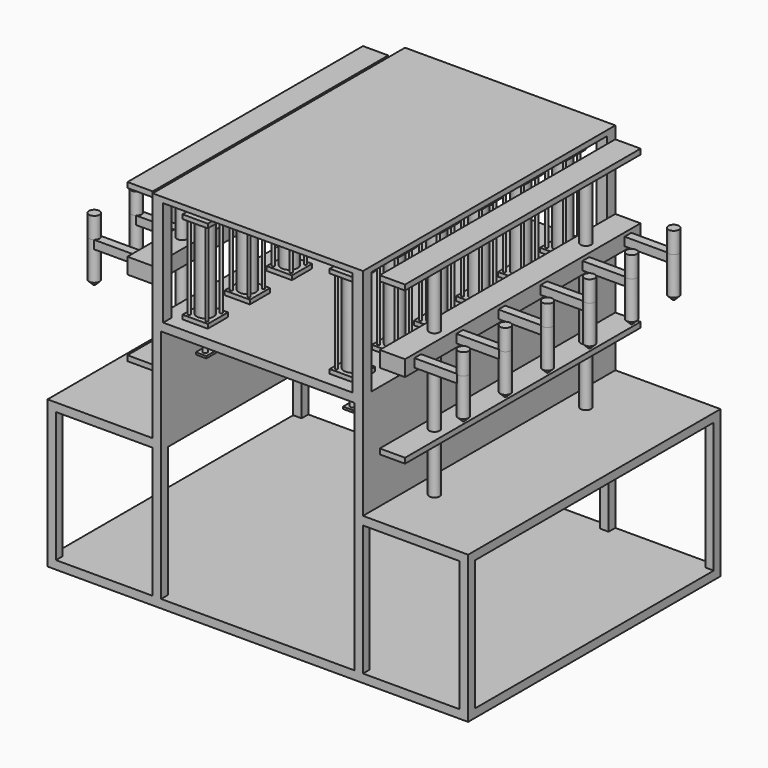
from build123d import *

# Parameters (mm, degrees)
F1_DEPTH       = 1500
F2_W           = 460
F2_H           = 620
F3_DEPTH       = 1500.001
F4_W           = 1420
F4_H           = 620
F5_DEPTH       = 2000.001
F6_W           = 120
F6_H           = 120
F7_DEPTH       = 20
F8_R           = 40
F9_DEPTH       = 400
F10_R          = 6
F11_DEPTH      = 400
F12_W          = 120
F12_H          = 120
F13_DEPTH      = 20
F14_R          = 11
F15_DEPTH      = 100
F16_W          = 50
F16_H          = 1300
F17_DEPTH      = 10
F18_R          = 25
F19_DEPTH      = 1000
F21_W          = 120
F21_H          = 1400
F22_DEPTH      = 25
F23_W          = 120
F23_H          = 1400
F24_DEPTH      = 25
F26_W          = 120
F26_H          = 1400
F27_DEPTH      = 75
F28_W          = 40
F28_H          = 40
F29_DEPTH      = 217.5
F30_R          = 25
F31_DEPTH      = 100
F31_DEPTH_BACK = 200
F32_SIZE       = 20
F33_W          = 50
F33_H          = 50
F34_DEPTH      = 500
F35_W          = 1000
F35_H          = 1500
F36_DEPTH      = 25


# Not quite as in the source:
# - a pattern or mirror of a feature is missing from the dataset's text; its kind, count and spacing are read off the source's solid


with BuildPart() as f1:
    # F0 (on Front) → F1 (new body)
    with BuildSketch(Plane.XZ):
        Polygon((-1000, 0), (0, 0), (0, 1200), (-500, 1200), (-500, 700), (-1000, 700), align=None)
        Polygon((0, 1200), (0, 0), (1000, 0), (1000, 700), (500, 700), (500, 1200), align=None)
    extrude(amount=F1_DEPTH)

    # F2 (on face) → F3 (cut, through all)
    with BuildSketch(Plane.XZ.offset(1500)):
        with Locations((-730, 350)):
            Rectangle(F2_W, F2_H)
        with Locations((730, 350)):
            Rectangle(F2_W, F2_H)
        Polygon((460, 1160), (-460, 1160), (-460, 660), (-460, 40), (460, 40), (460, 660), align=None)
    extrude(amount=-F3_DEPTH, mode=Mode.SUBTRACT)

    # F4 (on face) → F5 (cut, through all)
    with BuildSketch(Plane.YZ.offset(1000)):
        with Locations((-750, 350)):
            Rectangle(F4_W, F4_H)
    extrude(amount=-F5_DEPTH, mode=Mode.SUBTRACT)

    # F6 (on face) → F7 (join)
    with BuildSketch(Plane.XY.offset(1200)):
        with Locations((-350, -125)):
            Rectangle(F6_W, F6_H)
        with Locations((-350, -375)):
            Rectangle(F6_W, F6_H)
        with Locations((-350, -625)):
            Rectangle(F6_W, F6_H)
        with Locations((-350, -875)):
            Rectangle(F6_W, F6_H)
        with Locations((-350, -1125)):
            Rectangle(F6_W, F6_H)
        with Locations((-350, -1375)):
            Rectangle(F6_W, F6_H)
        with Locations((350, -125)):
            Rectangle(F6_W, F6_H)
        with Locations((350, -375)):
            Rectangle(F6_W, F6_H)
        with Locations((350, -625)):
            Rectangle(F6_W, F6_H)
        with Locations((350, -875)):
            Rectangle(F6_W, F6_H)
        with Locations((350, -1125)):
            Rectangle(F6_W, F6_H)
        with Locations((350, -1375)):
            Rectangle(F6_W, F6_H)
    extrude(amount=F7_DEPTH)

    # F8 (on face) → F9 (join)
    with BuildSketch(Plane.XY.offset(1220)):
        with Locations((-350, -1375)):
            Circle(F8_R)
        with Locations((-350, -1125)):
            Circle(F8_R)
        with Locations((-350, -875)):
            Circle(F8_R)
        with Locations((-350, -625)):
            Circle(F8_R)
        with Locations((-350, -375)):
            Circle(F8_R)
        with Locations((-350, -125)):
            Circle(F8_R)
        with Locations((350, -1375)):
            Circle(F8_R)
        with Locations((350, -1125)):
            Circle(F8_R)
        with Locations((350, -875)):
            Circle(F8_R)
        with Locations((350, -625)):
            Circle(F8_R)
        with Locations((350, -375)):
            Circle(F8_R)
        with Locations((350, -125)):
            Circle(F8_R)
    extrude(amount=F9_DEPTH)

    # F10 (on face) → F11 (join)
    with BuildSketch(Plane.XY.offset(1220)):
        with Locations((-307.5, -1332.5)):
            Circle(F10_R)
        with Locations((-392.5, -1332.5)):
            Circle(F10_R)
        with Locations((-307.5, -1417.5)):
            Circle(F10_R)
        with Locations((-392.5, -1417.5)):
            Circle(F10_R)
        with Locations((-307.5, -1082.5)):
            Circle(F10_R)
        with Locations((-392.5, -1082.5)):
            Circle(F10_R)
        with Locations((-392.5, -1167.5)):
            Circle(F10_R)
        with Locations((-307.5, -1167.5)):
            Circle(F10_R)
        with Locations((-307.5, -832.5)):
            Circle(F10_R)
        with Locations((-392.5, -832.5)):
            Circle(F10_R)
        with Locations((-392.5, -917.5)):
            Circle(F10_R)
        with Locations((-307.5, -917.5)):
            Circle(F10_R)
        with Locations((-307.5, -582.5)):
            Circle(F10_R)
        with Locations((-392.5, -582.5)):
            Circle(F10_R)
        with Locations((-392.5, -667.5)):
            Circle(F10_R)
        with Locations((-307.5, -667.5)):
            Circle(F10_R)
        with Locations((-307.5, -332.5)):
            Circle(F10_R)
        with Locations((-392.5, -332.5)):
            Circle(F10_R)
        with Locations((-392.5, -417.5)):
            Circle(F10_R)
        with Locations((-307.5, -417.5)):
            Circle(F10_R)
        with Locations((-307.5, -82.5)):
            Circle(F10_R)
        with Locations((-392.5, -82.5)):
            Circle(F10_R)
        with Locations((-392.5, -167.5)):
            Circle(F10_R)
        with Locations((-307.5, -167.5)):
            Circle(F10_R)
        with Locations((392.5, -1332.5)):
            Circle(F10_R)
        with Locations((307.5, -1332.5)):
            Circle(F10_R)
        with Locations((307.5, -1417.5)):
            Circle(F10_R)
        with Locations((392.5, -1417.5)):
            Circle(F10_R)
        with Locations((392.5, -1082.5)):
            Circle(F10_R)
        with Locations((307.5, -1082.5)):
            Circle(F10_R)
        with Locations((307.5, -1167.5)):
            Circle(F10_R)
        with Locations((392.5, -1167.5)):
            Circle(F10_R)
        with Locations((392.5, -832.5)):
            Circle(F10_R)
        with Locations((307.5, -832.5)):
            Circle(F10_R)
        with Locations((307.5, -917.5)):
            Circle(F10_R)
        with Locations((392.5, -917.5)):
            Circle(F10_R)
        with Locations((392.5, -582.5)):
            Circle(F10_R)
        with Locations((307.5, -582.5)):
            Circle(F10_R)
        with Locations((307.5, -667.5)):
            Circle(F10_R)
        with Locations((392.5, -667.5)):
            Circle(F10_R)
        with Locations((392.5, -332.5)):
            Circle(F10_R)
        with Locations((307.5, -332.5)):
            Circle(F10_R)
        with Locations((307.5, -417.5)):
            Circle(F10_R)
        with Locations((392.5, -417.5)):
            Circle(F10_R)
        with Locations((392.5, -82.5)):
            Circle(F10_R)
        with Locations((307.5, -82.5)):
            Circle(F10_R)
        with Locations((307.5, -167.5)):
            Circle(F10_R)
        with Locations((392.5, -167.5)):
            Circle(F10_R)
    extrude(amount=F11_DEPTH)

    # F12 (on face) → F13 (join)
    with BuildSketch(Plane.XY.offset(1620)):
        with Locations((-350, -1375)):
            Rectangle(F12_W, F12_H)
        with Locations((-350, -1125)):
            Rectangle(F12_W, F12_H)
        with Locations((-350, -875)):
            Rectangle(F12_W, F12_H)
        with Locations((-350, -625)):
            Rectangle(F12_W, F12_H)
        with Locations((-350, -375)):
            Rectangle(F12_W, F12_H)
        with Locations((-350, -125)):
            Rectangle(F12_W, F12_H)
        with Locations((350, -1375)):
            Rectangle(F12_W, F12_H)
        with Locations((350, -1125)):
            Rectangle(F12_W, F12_H)
        with Locations((350, -875)):
            Rectangle(F12_W, F12_H)
        with Locations((350, -625)):
            Rectangle(F12_W, F12_H)
        with Locations((350, -375)):
            Rectangle(F12_W, F12_H)
        with Locations((350, -125)):
            Rectangle(F12_W, F12_H)
    extrude(amount=F13_DEPTH)

    # F14 (on face) → F15 (join)
    with BuildSketch(Plane(origin=(0, 0, 1160), x_dir=(1, 0, 0), z_dir=(0, 0, -1))):
        with Locations((-350, 125)):
            Circle(F14_R)
        with Locations((-350, 375)):
            Circle(F14_R)
        with Locations((-350, 625)):
            Circle(F14_R)
        with Locations((-350, 875)):
            Circle(F14_R)
        with Locations((-350, 1125)):
            Circle(F14_R)
        with Locations((-350, 1375)):
            Circle(F14_R)
        with Locations((350, 125)):
            Circle(F14_R)
        with Locations((350, 375)):
            Circle(F14_R)
        with Locations((350, 625)):
            Circle(F14_R)
        with Locations((350, 875)):
            Circle(F14_R)
        with Locations((350, 1125)):
            Circle(F14_R)
        with Locations((350, 1375)):
            Circle(F14_R)
    extrude(amount=F15_DEPTH)

    # F16 (on face) → F17 (join)
    with BuildSketch(Plane(origin=(0, 0, 1060), x_dir=(1, 0, 0), z_dir=(0, 0, -1))):
        with Locations((-350, 750)):
            Rectangle(F16_W, F16_H)
        with Locations((350, 750)):
            Rectangle(F16_W, F16_H)
    extrude(amount=F17_DEPTH)

    # F18 (on face) → F19 (join)
    with BuildSketch(Plane.XY.offset(700)):
        with Locations((-600, -300)):
            Circle(F18_R)
        with Locations((600, -300)):
            Circle(F18_R)
        with Locations((-600, -1200)):
            Circle(F18_R)
        with Locations((600, -1200)):
            Circle(F18_R)
    extrude(amount=F19_DEPTH)

    # F21 (on offset) → F22 (join)
    with BuildSketch(Plane.XY.offset(950)):
        with Locations((-600, -750)):
            Rectangle(F21_W, F21_H)
        with Locations((600, -750)):
            Rectangle(F21_W, F21_H)
    extrude(amount=F22_DEPTH)

    # F23 (on face) → F24 (join)
    with BuildSketch(Plane.XY.offset(1700)):
        with Locations((-600, -750)):
            Rectangle(F23_W, F23_H)
        with Locations((600, -750)):
            Rectangle(F23_W, F23_H)
    extrude(amount=-F24_DEPTH)

    # F26 (on offset) → F27 (join)
    with BuildSketch(Plane.XY.offset(1312.5)):
        with Locations((-600, -750)):
            Rectangle(F26_W, F26_H)
        with Locations((600, -750)):
            Rectangle(F26_W, F26_H)
    extrude(amount=F27_DEPTH)

    # F28 (on face) → F29 (join)
    with BuildSketch(Plane(origin=(-660, 0, 0), x_dir=(0, -1, 0), z_dir=(-1, 0, 0))):
        with Locations((125, 1350)):
            Rectangle(F28_W, F28_H)
        with Locations((375, 1350)):
            Rectangle(F28_W, F28_H)
        with Locations((625, 1350)):
            Rectangle(F28_W, F28_H)
        with Locations((875, 1350)):
            Rectangle(F28_W, F28_H)
        with Locations((1125, 1350)):
            Rectangle(F28_W, F28_H)
        with Locations((1375, 1350)):
            Rectangle(F28_W, F28_H)
    f29 = extrude(amount=F29_DEPTH)

    # F29_copies: F29 across plane
    add(f29.mirror(Plane(origin=(0, 0, 0), x_dir=(0, 0, 1), z_dir=(1, 0, 0))))

    # F30 (on face) → F31 (join, two sides)
    with BuildSketch(Plane.XY.offset(1370)) as f31_sk:
        with Locations((-877.5, -125)):
            Circle(F30_R)
        with Locations((-877.5, -375)):
            Circle(F30_R)
        with Locations((-877.5, -625)):
            Circle(F30_R)
        with Locations((-877.5, -875)):
            Circle(F30_R)
        with Locations((-877.5, -1125)):
            Circle(F30_R)
        with Locations((-877.5, -1375)):
            Circle(F30_R)
        with Locations((877.5, -125)):
            Circle(F30_R)
        with Locations((877.5, -375)):
            Circle(F30_R)
        with Locations((877.5, -625)):
            Circle(F30_R)
        with Locations((877.5, -1125)):
            Circle(F30_R)
        with Locations((877.5, -1375)):
            Circle(F30_R)
        with Locations((877.5, -875)):
            Circle(F30_R)
    extrude(amount=F31_DEPTH)
    extrude(f31_sk.sketch, amount=-F31_DEPTH_BACK)

    # F32
    f32_edges = [f1.edges().sort_by_distance(p)[0] for p in [
        (-902.5, -1375, 1170),
        (-902.5, -1125, 1170),
        (-902.5, -875, 1170),
        (-902.5, -625, 1170),
        (-902.5, -375, 1170),
        (-902.5, -125, 1170),
        (852.5, -1375, 1170),
        (852.5, -1125, 1170),
        (852.5, -875, 1170),
        (852.5, -625, 1170),
        (852.5, -125, 1170),
        (852.5, -375, 1170),
    ]]
    chamfer(f32_edges, length=F32_SIZE)

    # F33 (on face) → F34 (join)
    with BuildSketch(Plane.XY.offset(1200)):
        with Locations((-475, -25)):
            Rectangle(F33_W, F33_H)
        with Locations((475, -25)):
            Rectangle(F33_W, F33_H)
        with Locations((-475, -1475)):
            Rectangle(F33_W, F33_H)
        with Locations((475, -1475)):
            Rectangle(F33_W, F33_H)
    extrude(amount=F34_DEPTH)

    # F35 (on face) → F36 (join)
    with BuildSketch(Plane.XY.offset(1700)):
        with Locations((0, -750)):
            Rectangle(F35_W, F35_H)
    extrude(amount=F36_DEPTH)


solid = f1.part
